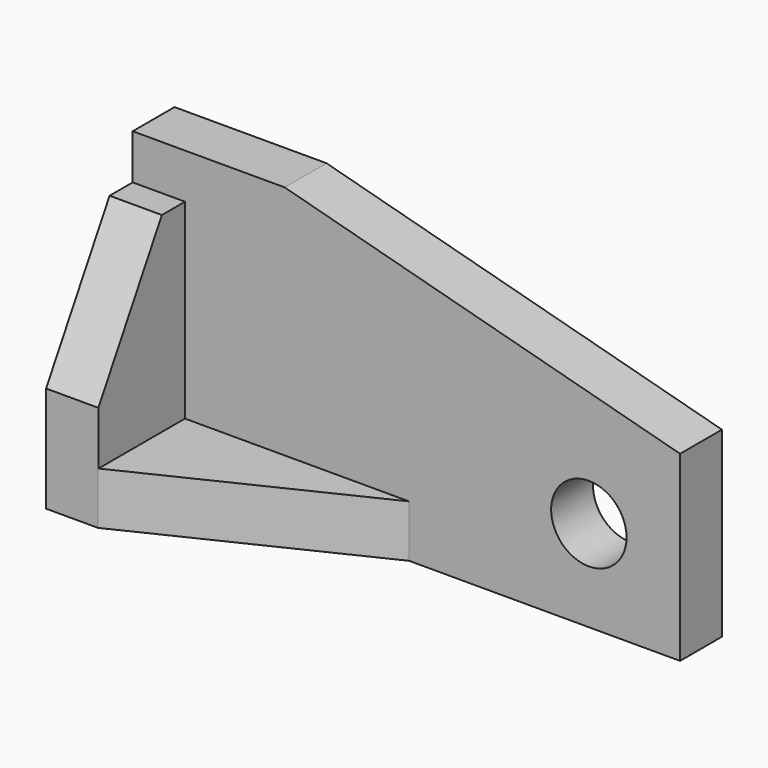
from build123d import *

# Parameters (mm, degrees)
F0_R        = 7.874
F1_DEPTH    = 10.922
F0_W        = 52.578
F0_H        = 10.922
F2_DEPTH    = 33.528
F3_SIZE2    = 22.1192058352
F3_SIZE     = 82.55
F4_T4_DEPTH = 283.7447130195
F5_SIZE2    = 16.5711074263
F5_SIZE     = 28.702


# Not quite as in the source:
# - a fillet or chamfer that OpenCascade refuses, or shapes differently, is made with other operations: its cross-section is extruded or revolved along the edge and cut away or added


with BuildPart() as f1:
    # F0 (on Front) → F1 (new body)
    with BuildSketch(Plane.XZ):
        Polygon((56.9204140842, 23.2569413837), (-57.3795859158, 23.2569413837), (-57.3795859158, 13.8589413837), (-46.4575859158, 13.8589413837), (-46.4575859158, -26.0190586163), (6.1204140842, -26.0190586163), (6.1204140842, -36.9410586163), (56.9204140842, -36.9410586163), align=None)
        with Locations((37.8704140842, -17.8910586163)):
            Circle(F0_R, mode=Mode.SUBTRACT)
    extrude(amount=F1_DEPTH)

    # F0 (on Front) → F2 (join)
    with BuildSketch(Plane.XZ):
        Polygon((-46.4575859158, 13.8589413837), (-57.3795859158, 13.8589413837), (-57.3795859158, -36.9410586163), (-46.4575859158, -36.9410586163), (-46.4575859158, -26.0190586163), align=None)
        with Locations((-20.1685859158, -31.4800586163)):
            Rectangle(F0_W, F0_H)
    extrude(amount=F2_DEPTH)

    # F3
    f3_edges = [f1.edges().sort_by_distance(p)[0] for p in [
        (56.920414, -5.461, 23.256941),
    ]]
    f3_side = f1.faces().sort_by_distance((-0.229586, -5.461, 23.256941))[0]
    chamfer(f3_edges, length=F3_SIZE, length2=F3_SIZE2, reference=f3_side)

    # F4: chamfer of 25.4 x 52.6596501835 on 1 edges, made by hand


with BuildPart() as f4_tool2:
    # F4_s3 → F4_t4 (new body)
    with BuildSketch(Plane.XY.offset(-173.3524151261)):
        Polygon((-46.5392360993, -33.528), (6.1204140842, -8.128), (6.1204140842, -33.528), align=None)
    extrude(amount=F4_T4_DEPTH)

    split(bisect_by=Plane.XZ.offset(10.922), keep=Keep.TOP)


with BuildPart() as f1_1:
    add(f1.part)

    # F4_t1: cut F4_tool2
    add(f4_tool2.part, mode=Mode.SUBTRACT)

    # F5
    f5_edges = [f1_1.edges().sort_by_distance(p)[0] for p in [
        (-51.959411, -33.528, 13.858941),
    ]]
    f5_side = f1_1.faces().sort_by_distance((-51.959411, -33.528, -11.541059))[0]
    chamfer(f5_edges, length=F5_SIZE, length2=F5_SIZE2, reference=f5_side)


solid = f1_1.part
